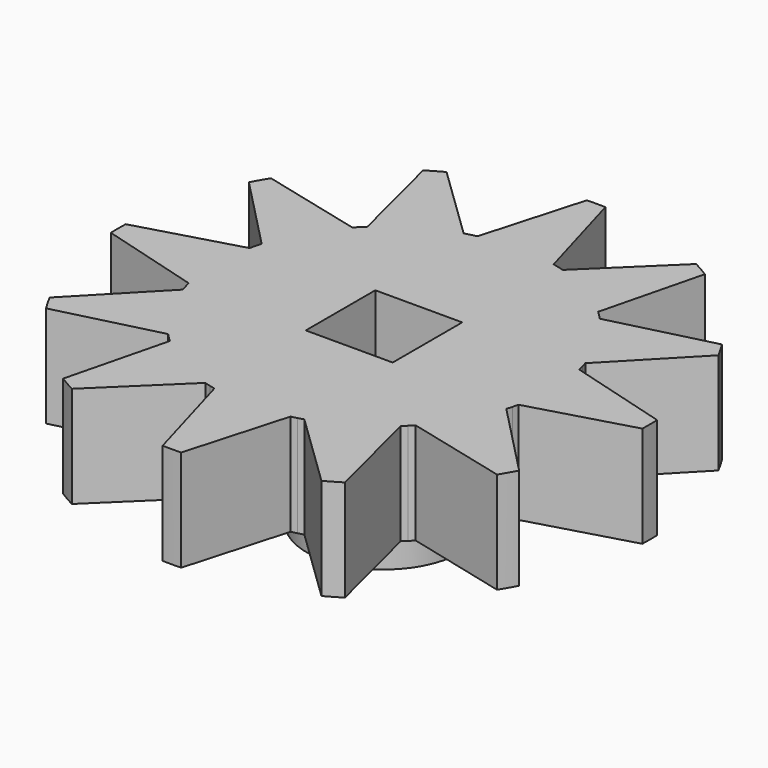
from build123d import *

# Parameters (mm, degrees)
F0_R            = 11
F1_DEPTH        = 4.2
F3_DEPTH        = 25
F3_COPIES_COUNT = 12
F5_R            = 3.2
F6_DEPTH        = 3
F7_W            = 3.6
F7_H            = 3.6
F8_DEPTH        = 7.201


# Not quite as in the source:
# - a pattern or mirror of a feature is missing from the dataset's text; its kind, count and spacing are read off the source's solid


with BuildPart() as f1:
    # F0 (on Top) → F1 (new body)
    with BuildSketch(Plane.XY):
        Circle(F0_R)
    extrude(amount=F1_DEPTH)

    # F2 (on face) → F3 (cut)
    with BuildSketch(Plane(origin=(0, 0, 0), x_dir=(1, 0, 0), z_dir=(0, 0, -1))):
        with BuildLine():
            ThreePointArc((-6.8188061736, 1.5823660658), (-6.7901515407, 1.7011296406), (-6.7594285619, 1.8193750347))
            Line((-6.7594285619, 1.8193750347), (-10.6219591686, 2.8590179117))
            ThreePointArc((-10.6219591686, 2.8590179117), (-10.8773296979, 1.6381998176), (-10.9928581369, 0.3963205537))
            Line((-10.9928581369, 0.3963205537), (-6.8188061736, 1.5823660658))
        make_face()
        with BuildLine():
            Line((-10.6219591686, 2.8590179117), (-6.7594285619, 1.8193750347))
            ThreePointArc((-6.7594285619, 1.8193750347), (-6.7266465956, 1.9370662297), (-6.6918156276, 2.0541673754))
            Line((-6.6918156276, 2.0541673754), (-9.7065799497, 5.1751623821))
            ThreePointArc((-9.7065799497, 5.1751623821), (-10.2300296663, 4.0430796464), (-10.6219591686, 2.8590179117))
        make_face()
    f3 = extrude(amount=-F3_DEPTH, mode=Mode.SUBTRACT)

    # F3_copies: F3 ×12 about axis
    f3_copies_axis = Axis((0, 0, 0), (0, 0, 1))
    for i in range(1, F3_COPIES_COUNT):
        add(f3.rotate(f3_copies_axis, i * 360 / F3_COPIES_COUNT), mode=Mode.SUBTRACT)

    # F5 (on face) → F6 (join)
    with BuildSketch(Plane(origin=(0, 0, 0), x_dir=(1, 0, 0), z_dir=(0, 0, -1))):
        Circle(F5_R)
    extrude(amount=F6_DEPTH)

    # F7 (on face) → F8 (cut, through all)
    with BuildSketch(Plane(origin=(0, 0, -3), x_dir=(1, 0, 0), z_dir=(0, 0, -1))):
        Rectangle(F7_W, F7_H)
    extrude(amount=-F8_DEPTH, mode=Mode.SUBTRACT)


solid = f1.part
